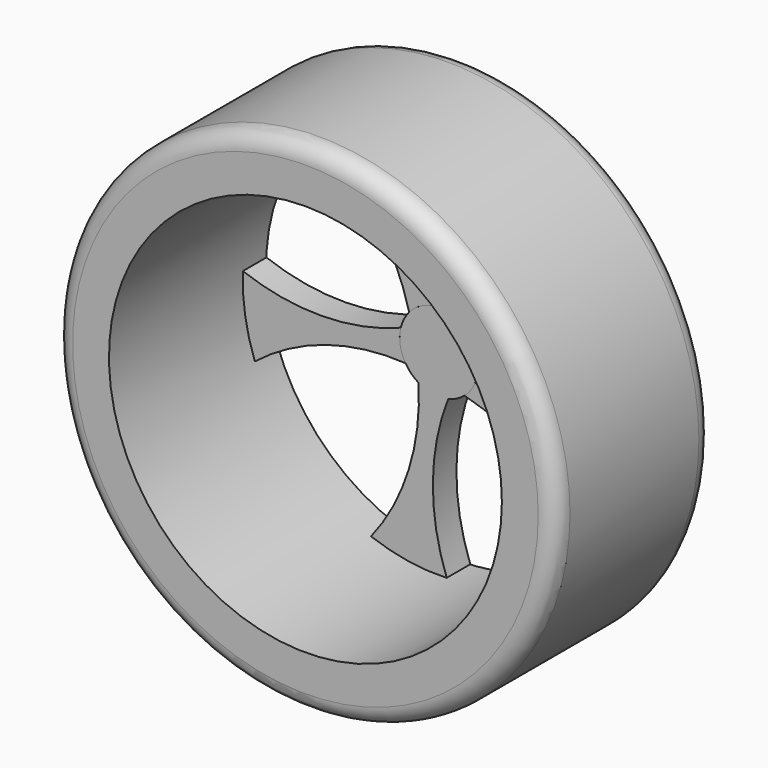
from build123d import *

# Parameters (mm, degrees)
F0_R     = 27.305
F1_DEPTH = 25.4
F2_DEPTH = 3.81
F3_DEPTH = 3.81
F0_R_2   = 32.385
F4_DEPTH = 25.4
F5_R     = 2.286


with BuildPart() as f1:
    # F0 (on Front) → F1 (new body)
    with BuildSketch(Plane.XZ):
        Circle(F0_R)
        with BuildLine():
            ThreePointArc((0, 25.4), (17.9605122421, 17.9605122421), (25.4, 0))
            ThreePointArc((25.4, 0), (-17.9605122421, -17.9605122421), (0, 25.4))
        make_face(mode=Mode.SUBTRACT)
    extrude(amount=F1_DEPTH)

    # F0 (on Front) → F4 (join)
    with BuildSketch(Plane.XZ):
        Circle(F0_R_2)
        Circle(F0_R, mode=Mode.SUBTRACT)
    extrude(amount=F4_DEPTH)

    # F5
    f5_edges = [f1.edges().sort_by_distance(p)[0] for p in [
        (-32.385, 0, 0),
        (-32.385, -25.4, 0),
    ]]
    fillet(f5_edges, radius=F5_R)


with BuildPart() as f2:
    # F0 (on Front) → F2 (new body)
    with BuildSketch(Plane.XZ):
        with BuildLine():
            ThreePointArc((4.6943420121, 1.9469076959), (11.7768309148, 9.5402464113), (21.1050706762, 14.1014288083))
            ThreePointArc((21.1050706762, 14.1014288083), (19.6204327638, 16.1017497715), (17.947313904, 17.947313904))
            ThreePointArc((17.947313904, 17.947313904), (16.1014099509, 19.6203250282), (14.1007988537, 21.1048730615))
            ThreePointArc((14.1007988537, 21.1048730615), (9.5399900472, 11.7767988623), (1.9471382686, 4.694246561))
            ThreePointArc((1.9471382686, 4.694246561), (2.8248144406, 4.2253038625), (3.5940705708, 3.5940608637))
            ThreePointArc((3.5940705708, 3.5940608637), (4.225376988, 2.8247049807), (4.6943420121, 1.9469076959))
        make_face()
        with BuildLine():
            ThreePointArc((24.4307833241, -6.8888302352), (14.14792832, -5.4336738514), (5.0642555877, -0.3996419851))
            ThreePointArc((5.0642555877, -0.3996419851), (4.5262563388, -2.3063828671), (3.2998221317, -3.862327313))
            ThreePointArc((3.2998221317, -3.862327313), (12.7127227114, -8.2524534489), (19.9346977885, -15.716968222))
            ThreePointArc((19.9346977885, -15.716968222), (22.5923186543, -11.5114934038), (24.4307833241, -6.8888302352))
        make_face()
        with BuildLine():
            ThreePointArc((-3.8621651693, 3.3000119059), (-2.3061604636, 4.526369659), (-0.3993931489, 5.0642752183))
            ThreePointArc((-0.3993931489, 5.0642752183), (-5.4341382858, 14.1487260117), (-6.8893071571, 24.4326157606))
            ThreePointArc((-6.8893071571, 24.4326157606), (-11.5217587117, 22.6129744405), (-15.7157660774, 19.9332348715))
            ThreePointArc((-15.7157660774, 19.9332348715), (-8.2520810905, 12.7118781046), (-3.8621651693, 3.3000119059))
        make_face()
        with BuildLine():
            ThreePointArc((-1.5809043391, -4.8277468704), (-0.2058216404, -5.0761626418), (1.1848589263, -4.939889442))
            ThreePointArc((1.1848589263, -4.939889442), (-0.2058081178, -5.0758291335), (-1.5809043391, -4.8277468704))
        make_face()
        with BuildLine():
            ThreePointArc((0.9978603482, -25.3638212927), (-0.7957806377, -15.1345769828), (1.1848589263, -4.939889442))
            ThreePointArc((1.1848589263, -4.939889442), (-0.2058216404, -5.0761626418), (-1.5809043391, -4.8277468704))
            ThreePointArc((-1.5809043391, -4.8277468704), (-2.1317168887, -4.6110933064), (-2.653590442, -4.3318421186))
            ThreePointArc((-2.653590442, -4.3318421186), (-3.9201022654, -14.6406661355), (-8.7875646495, -23.8158345128))
            ThreePointArc((-8.7875646495, -23.8158345128), (-3.9710774773, -25.0716777648), (0.9978603482, -25.3638212927))
        make_face()
        with BuildLine():
            ThreePointArc((-4.3319724994, -2.6533775907), (-5.0174761344, -0.794563789), (-4.9398312171, 1.1851016499))
            ThreePointArc((-4.9398312171, 1.1851016499), (-15.1354791508, -0.7959758408), (-25.3657114203, 0.9979730226))
            ThreePointArc((-25.3657114203, 0.9979730226), (-25.067740133, -3.9702254045), (-23.814071713, -8.7868734083))
            ThreePointArc((-23.814071713, -8.7868734083), (-14.6397478017, -3.9200091294), (-4.3319724994, -2.6533775907))
        make_face()
        with BuildLine():
            ThreePointArc((-2.653590442, -4.3318421186), (-2.1317168887, -4.6110933064), (-1.5809043391, -4.8277468704))
            ThreePointArc((-1.5809043391, -4.8277468704), (-2.1318038089, -4.6106814204), (-2.6536484216, -4.3308853596))
            ThreePointArc((-2.6536484216, -4.3308853596), (-2.6536194278, -4.3313637388), (-2.653590442, -4.3318421186))
        make_face()
    extrude(amount=F2_DEPTH)

    # F0 (on Front) → F3 (join)
    with BuildSketch(Plane.XZ):
        with BuildLine():
            ThreePointArc((5.0642555877, -0.3996419851), (5.0760622509, -0.1999759972), (5.07999984, 0))
            ThreePointArc((5.07999984, 0), (4.9814434579, 0.990970805), (4.6924772139, 1.9439844496))
            ThreePointArc((4.6924772139, 1.9439844496), (4.5453190283, 2.2675494992), (4.3760141266, 2.5800966528))
            ThreePointArc((4.3760141266, 2.5800966528), (4.0169149714, 3.1097897818), (3.5940705708, 3.5901330207))
            ThreePointArc((3.5940705708, 3.5901330207), (1.9450231546, 4.692046096), (1.37204e-05, 5.0799998399))
            ThreePointArc((1.37204e-05, 5.0799998399), (-0.1998444343, 5.0760674322), (-0.3993931489, 5.0642752183))
            ThreePointArc((-0.3993931489, 5.0642752183), (-0.3990885143, 5.0639052384), (-0.3987838736, 5.0635352636))
            ThreePointArc((-0.3987838736, 5.0635352636), (-2.3055656836, 4.5256348971), (-3.8621651693, 3.3000119059))
            ThreePointArc((-3.8621651693, 3.3000119059), (-4.5262563388, 2.3063828671), (-4.9398312171, 1.1851016499))
            ThreePointArc((-4.9398312171, 1.1851016499), (-4.9393852081, 1.1852770445), (-4.9389392019, 1.1854524465))
            ThreePointArc((-4.9389392019, 1.1854524465), (-5.0168667916, -0.7942683785), (-4.3319724994, -2.6533775907))
            ThreePointArc((-4.3319724994, -2.6533775907), (-3.5921905844, -3.5920140839), (-2.653590442, -4.3318421186))
            ThreePointArc((-2.653590442, -4.3318421186), (-2.6536194278, -4.3313637388), (-2.6536484216, -4.3308853596))
            ThreePointArc((-2.6536484216, -4.3308853596), (-2.1318038089, -4.6106814204), (-1.5809043391, -4.8277468704))
            ThreePointArc((-1.5809043391, -4.8277468704), (-0.2058081178, -5.0758291335), (1.1848589263, -4.939889442))
            ThreePointArc((1.1848589263, -4.939889442), (2.3061604635, -4.5263696591), (3.2998221317, -3.862327313))
            ThreePointArc((3.2998221317, -3.862327313), (3.2993582084, -3.8622070527), (3.2988942831, -3.8620868001))
            ThreePointArc((3.2988942831, -3.8620868001), (4.5249044889, -2.3059143186), (5.0642555877, -0.3996419851))
        make_face()
    extrude(amount=F3_DEPTH)


solid = Compound([f1.part, f2.part])
